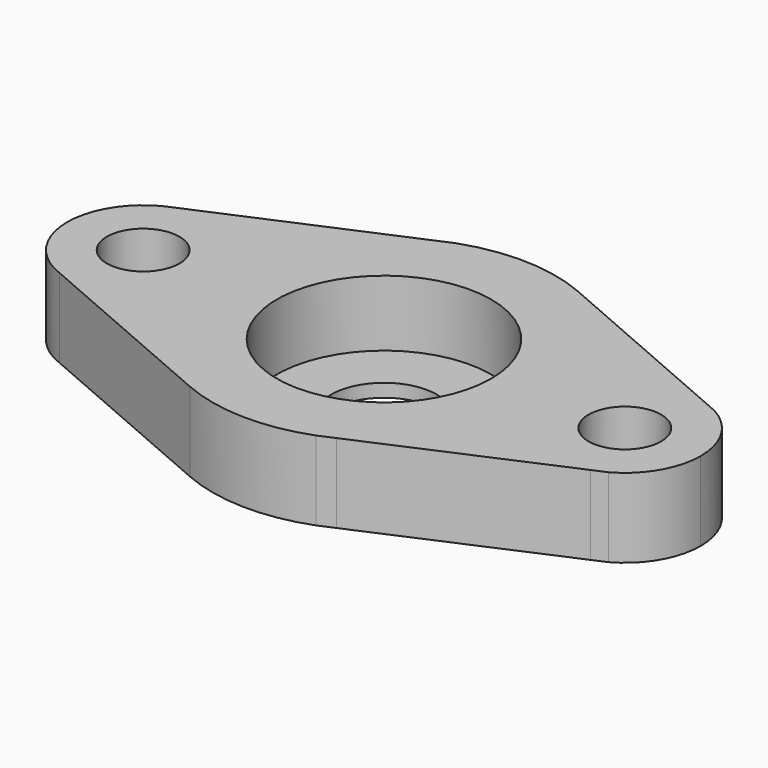
from build123d import *

# Parameters (mm, degrees)
F0_R     = 2.75
F0_R_2   = 4
F1_DEPTH = 6
F2_R     = 8.125
F2_R_2   = 4
F3_DEPTH = 5


# Not quite as in the source:
# - a feature names something its author has since deleted; it is built from what else it names


with BuildPart() as f1:
    # F0 (on Top) → F1 (new body)
    with BuildSketch(Plane.XY):
        with BuildLine():
            ThreePointArc((20.0822139412, 5.4502744952), (15.7589539647, 5.182392271), (12.8493150685, 1.9736013454))
            ThreePointArc((12.8493150685, 1.9736013454), (12.9622740268, 0.9896727008), (13, 0))
            ThreePointArc((13, 0), (12.9622740268, -0.9896727008), (12.8493150685, -1.9736013454))
            ThreePointArc((12.8493150685, -1.9736013454), (15.7262122641, -5.1665264409), (20.0130954241, -5.4730242577))
            Line((20.0130954241, -5.4730242577), (21.0412591059, -5.0270640143))
            ThreePointArc((21.0412591059, -5.0270640143), (23.2054131946, -2.9165699153), (24, 0))
            ThreePointArc((24, 0), (23.1883419046, 2.9453826972), (20.982511571, 5.0592371474))
            Line((20.982511571, 5.0592371474), (20.0822139412, 5.4502744952))
        make_face()
        with Locations((18.25, 0)):
            Circle(F0_R, mode=Mode.SUBTRACT)
        with BuildLine():
            Line((20.0822139412, 5.4502744952), (5.2758693561, 11.8812963323))
            ThreePointArc((5.2758693561, 11.8812963323), (10.328174214, 7.8948601891), (12.8493150685, 1.9736013454))
            ThreePointArc((12.8493150685, 1.9736013454), (15.7589539647, 5.182392271), (20.0822139412, 5.4502744952))
        make_face()
        with BuildLine():
            ThreePointArc((13, 0), (12.9622740268, 0.9896727008), (12.8493150685, 1.9736013454))
            ThreePointArc((12.8493150685, 1.9736013454), (12.5, 0), (12.8493150685, -1.9736013454))
            ThreePointArc((12.8493150685, -1.9736013454), (12.9622740268, -0.9896727008), (13, 0))
        make_face()
        with BuildLine():
            ThreePointArc((20.0130954241, -5.4730242577), (15.7262122641, -5.1665264409), (12.8493150685, -1.9736013454))
            ThreePointArc((12.8493150685, -1.9736013454), (10.4831727002, -7.6878534154), (5.7442785493, -11.6620437295))
            Line((5.7442785493, -11.6620437295), (20.0130954241, -5.4730242577))
        make_face()
        with BuildLine():
            Line((5.2758693561, 11.8812963323), (5.0818351063, 11.9655736157))
            ThreePointArc((5.0818351063, 11.9655736157), (0.4274688612, 12.9929700366), (-4.2843620194, 12.273721607))
            Line((-4.2843620194, 12.273721607), (-5.9821590265, 11.5418271249))
            ThreePointArc((-5.9821590265, 11.5418271249), (-10.5614317348, 7.5799841498), (-12.8493150685, 1.9736013454))
            ThreePointArc((-12.8493150685, 1.9736013454), (-12.588002192, 1.0021381252), (-12.5, 0))
            ThreePointArc((-12.5, 0), (-12.588002192, -1.0021381252), (-12.8493150685, -1.9736013454))
            ThreePointArc((-12.8493150685, -1.9736013454), (-10.2925346971, -7.9412675001), (-5.1687008476, -11.9283079918))
            ThreePointArc((-5.1687008476, -11.9283079918), (-0.3123803464, -12.9962463242), (4.589640736, -12.1628614197))
            Line((4.589640736, -12.1628614197), (5.7442785493, -11.6620437295))
            ThreePointArc((5.7442785493, -11.6620437295), (10.4831727002, -7.6878534154), (12.8493150685, -1.9736013454))
            ThreePointArc((12.8493150685, -1.9736013454), (12.5, 0), (12.8493150685, 1.9736013454))
            ThreePointArc((12.8493150685, 1.9736013454), (10.328174214, 7.8948601891), (5.2758693561, 11.8812963323))
        make_face()
        Circle(F0_R_2, mode=Mode.SUBTRACT)
        with BuildLine():
            ThreePointArc((-12.8493150685, -1.9736013454), (-13, 0), (-12.8493150685, 1.9736013454))
            ThreePointArc((-12.8493150685, 1.9736013454), (-15.8411768162, 5.2211177797), (-20.2535684755, 5.3896394466))
            ThreePointArc((-20.2535684755, 5.3896394466), (-23.9999641766, 0.020296977), (-20.2915681825, -5.3753603932))
            ThreePointArc((-20.2915681825, -5.3753603932), (-15.8596218943, -5.229588178), (-12.8493150685, -1.9736013454))
        make_face()
        with Locations((-18.25, 0)):
            Circle(F0_R, mode=Mode.SUBTRACT)
        with BuildLine():
            ThreePointArc((-12.5, 0), (-12.588002192, 1.0021381252), (-12.8493150685, 1.9736013454))
            ThreePointArc((-12.8493150685, 1.9736013454), (-13, 0), (-12.8493150685, -1.9736013454))
            ThreePointArc((-12.8493150685, -1.9736013454), (-12.588002192, -1.0021381252), (-12.5, 0))
        make_face()
        with BuildLine():
            ThreePointArc((-12.8493150685, 1.9736013454), (-10.5614317348, 7.5799841498), (-5.9821590265, 11.5418271249))
            Line((-5.9821590265, 11.5418271249), (-20.2535684755, 5.3896394466))
            ThreePointArc((-20.2535684755, 5.3896394466), (-15.8411768162, 5.2211177797), (-12.8493150685, 1.9736013454))
        make_face()
        with BuildLine():
            ThreePointArc((-5.1687008476, -11.9283079918), (-10.2925346971, -7.9412675001), (-12.8493150685, -1.9736013454))
            ThreePointArc((-12.8493150685, -1.9736013454), (-15.8596218943, -5.229588178), (-20.2915681825, -5.3753603932))
            Line((-20.2915681825, -5.3753603932), (-5.1687008476, -11.9283079918))
        make_face()
    extrude(amount=F1_DEPTH)

    # F2 (on face) → F3 (cut)
    with BuildSketch(Plane.XY.offset(6)):
        Circle(F2_R)
        Circle(F2_R_2, mode=Mode.SUBTRACT)
    extrude(amount=-F3_DEPTH, mode=Mode.SUBTRACT)


solid = f1.part
